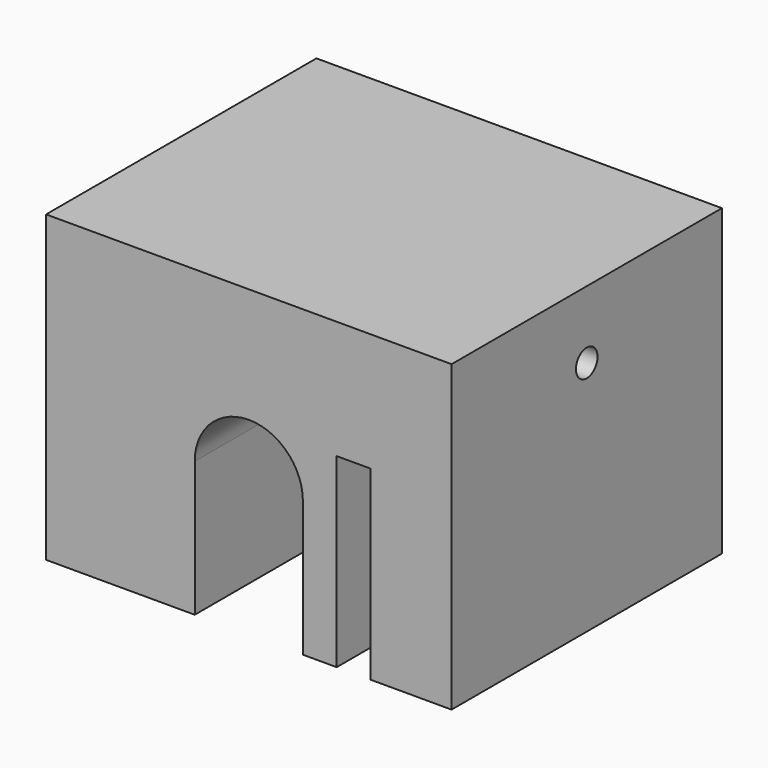
from build123d import *

# Parameters (mm, degrees)
F1_DEPTH = 10
F3_DEPTH = 0.5
F4_R     = 0.3
F5_W     = 1
F5_H     = 10
F6_DEPTH = 5.5
F7_R     = 0.4
F8_DEPTH = 12.001


# Not quite as in the source:
# - a feature names something its author has since deleted; it is built from what else it names


with BuildPart() as f1:
    # F0 (on Front) → F1 (new body)
    with BuildSketch(Plane.XZ):
        with BuildLine():
            Line((-6, 9), (-6, 0))
            Line((-6, 0), (-1.6, 0))
            Line((-1.6, 0), (-1.6, 4))
            ThreePointArc((-1.6, 4), (0, 5.6), (1.6, 4))
            Line((1.6, 4), (1.6, 0))
            Line((1.6, 0), (6, 0))
            Line((6, 0), (6, 9))
            Line((6, 9), (-6, 9))
        make_face()
    extrude(amount=F1_DEPTH)

    # F2 (on face) → F3 (join)
    with BuildSketch(Plane(origin=(1.6, 0, 0), x_dir=(0, -1, 0), z_dir=(-1, 0, 0))):
        Polygon((5.1838214056, 6), (3, 0), (3.7, 0), (5.8838214056, 6), align=None)
        Polygon((6, 0), (6.7, 0), (8.8838214056, 6), (8.1838214056, 6), align=None)
    extrude(amount=F3_DEPTH)

    # F4
    f4_edges = [f1.edges().sort_by_distance(p)[0] for p in [
        (1.1, -3.939388, 2.580948),
        (1.1, -4.639388, 2.580948),
        (1.1, -6.939388, 2.580948),
        (1.1, -7.639388, 2.580948),
    ]]
    fillet(f4_edges, radius=F4_R)

    # F5 (on face) → F6 (cut)
    with BuildSketch(Plane(origin=(0, 0, 0), x_dir=(1, 0, 0), z_dir=(0, 0, -1))):
        with Locations((3.1, 5)):
            Rectangle(F5_W, F5_H)
    extrude(amount=-F6_DEPTH, mode=Mode.SUBTRACT)

    # F7 (on face) → F8 (cut, through all)
    with BuildSketch(Plane(origin=(-6, 0, 0), x_dir=(0, -1, 0), z_dir=(-1, 0, 0))):
        with Locations((5, 7)):
            Circle(F7_R)
    extrude(amount=-F8_DEPTH, mode=Mode.SUBTRACT)


solid = f1.part
